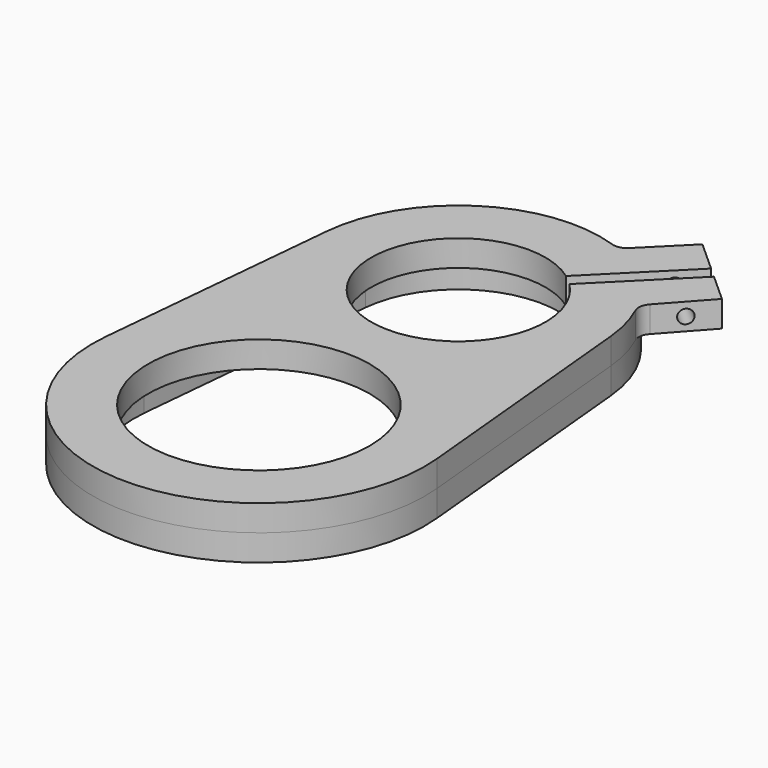
from build123d import *

# Parameters (mm, degrees)
F3_R      = 4.7625
F3_R_2    = 50.8
F4_DEPTH  = 11.9888
F5_R      = 3.175
F6_DEPTH  = 133.893314743
F8_DEPTH  = 11.9888
F10_DEPTH = 6.35
F11_DEPTH = 6.35
F12_DEPTH = 6.35


# Not quite as in the source:
# - a variable given as a bare number and used for a length is read in inches; the dataset says mm whatever the document's units were


with BuildPart() as f4:
    # F3 (on Top) → F4 (new body)
    with BuildSketch(Plane.XY):
        with BuildLine():
            ThreePointArc((28.2843044815, 64.8573104526), (-25.9422769004, 6.1262979516), (23.4354987006, 68.9887607928))
            Line((23.4354987006, 68.9887607928), (60.3862498519, 105.9395119442))
            Line((60.3862498519, 105.9395119442), (46.2066900189, 118.7007204743))
            Line((46.2066900189, 118.7007204743), (27.5367774821, 100.0308079375))
            ThreePointArc((27.5367774821, 100.0308079375), (24.4893412706, 98.3369938712), (21.0069821329, 98.5074297537))
            ThreePointArc((21.0069821329, 98.5074297537), (-35.5438535466, 91.4710990406), (-65.1074486079, 42.7525110788))
            Line((-65.1074486079, 42.7525110788), (-75.8590828523, -70.5270253622))
            ThreePointArc((-75.8590828523, -70.5270253622), (0, -153.9269940288), (75.8590828523, -70.5270253622))
            Line((75.8590828523, -70.5270253622), (65.1074486079, 42.7525110788))
            ThreePointArc((65.1074486079, 42.7525110788), (63.1878642435, 53.4389467972), (59.5267335018, 63.6605334739))
            ThreePointArc((59.5267335018, 63.6605334739), (59.0305262413, 67.2575870183), (60.5864824449, 70.5384430254))
            Line((60.5864824449, 70.5384430254), (78.0995628634, 89.9980240728))
            Line((78.0995628634, 89.9980240728), (65.1127697963, 101.6857757674))
            Line((65.1127697963, 101.6857757674), (28.2843044815, 64.8573104526))
        make_face()
        with Locations((0, -141.2269940288)):
            Circle(F3_R, mode=Mode.SUBTRACT)
        with Locations((-63.215902377, -71.72702014)):
            Circle(F3_R, mode=Mode.SUBTRACT)
        with Locations((0, -77.7269940288)):
            Circle(F3_R_2, mode=Mode.SUBTRACT)
        with Locations((63.215902377, -71.72702014)):
            Circle(F3_R, mode=Mode.SUBTRACT)
        with Locations((-57.8400852547, -15.0872519195)):
            Circle(F3_R, mode=Mode.SUBTRACT)
        with Locations((-52.4642681325, 41.552516301)):
            Circle(F3_R, mode=Mode.SUBTRACT)
        with Locations((57.8400852547, -15.0872519195)):
            Circle(F3_R, mode=Mode.SUBTRACT)
        with Locations((52.700047, 36.5730059712)):
            Circle(F3_R, mode=Mode.SUBTRACT)
        with Locations((-52.4642681325, 41.552516301)):
            Circle(F3_R)
        with Locations((52.700047, 36.5730059712)):
            Circle(F3_R)
        with Locations((57.8400852547, -15.0872519195)):
            Circle(F3_R)
        with Locations((63.215902377, -71.72702014)):
            Circle(F3_R)
        with Locations((0, -141.2269940288)):
            Circle(F3_R)
        with Locations((-63.215902377, -71.72702014)):
            Circle(F3_R)
        with Locations((-57.8400852547, -15.0872519195)):
            Circle(F3_R)
    extrude(amount=F4_DEPTH)

    # F5 (on face) → F6 (cut, through all)
    with BuildSketch(Plane(origin=(-1.6001270702, 1.4400697524, 0), x_dir=(0.6689532824, 0.7433044504, 0), z_dir=(0.7433044504, -0.6689532824, 0))):
        with Locations((106.0509778379, 5.9944)):
            Circle(F5_R)
    extrude(amount=-F6_DEPTH, mode=Mode.SUBTRACT)

    # F3 (on Top) → F10 (cut)
    with BuildSketch(Plane.XY):
        with Locations((-63.215902377, -71.72702014)):
            Circle(F3_R)
        with Locations((0, -141.2269940288)):
            Circle(F3_R)
        with Locations((63.215902377, -71.72702014)):
            Circle(F3_R)
        with Locations((57.8400852547, -15.0872519195)):
            Circle(F3_R)
        with Locations((52.700047, 36.5730059712)):
            Circle(F3_R)
        with Locations((-57.8400852547, -15.0872519195)):
            Circle(F3_R)
        with Locations((-52.4642681325, 41.552516301)):
            Circle(F3_R)
    extrude(amount=F10_DEPTH, mode=Mode.SUBTRACT)


with BuildPart() as f8:
    # F7 (on Top) → F8 (new body)
    with BuildSketch(Plane.XY):
        with BuildLine():
            Line((-65.1074486079, 42.7525110788), (-75.8590828523, -70.5270253622))
            ThreePointArc((-75.8590828523, -70.5270253622), (0, -153.9269940288), (75.8590828523, -70.5270253622))
            Line((75.8590828523, -70.5270253622), (65.1074486079, 42.7525110788))
            ThreePointArc((65.1074486079, 42.7525110788), (0, 101.9730529712), (-65.1074486079, 42.7525110788))
        make_face()
        with BuildLine():
            ThreePointArc((69.5374926147, -71.1270227511), (0, -147.5769940288), (-69.5374926147, -71.1270227511))
            Line((-69.5374926147, -71.1270227511), (-58.7858583702, 42.1525136899))
            ThreePointArc((-58.7858583702, 42.1525136899), (0, 95.6230529712), (58.7858583702, 42.1525136899))
            Line((58.7858583702, 42.1525136899), (69.5374926147, -71.1270227511))
        make_face(mode=Mode.SUBTRACT)
        with BuildLine():
            Line((-58.7858583702, 42.1525136899), (-69.5374926147, -71.1270227511))
            ThreePointArc((-69.5374926147, -71.1270227511), (0, -147.5769940288), (69.5374926147, -71.1270227511))
            Line((69.5374926147, -71.1270227511), (58.7858583702, 42.1525136899))
            ThreePointArc((58.7858583702, 42.1525136899), (0, 95.6230529712), (-58.7858583702, 42.1525136899))
        make_face()
        with BuildLine():
            ThreePointArc((-4.7591501891, -141.0484002788), (-46.9747184236, -120.4543369023), (-63.487789177, -76.4817529209))
            ThreePointArc((-63.487789177, -76.4817529209), (-67.9646903624, -71.3658845431), (-62.7656453711, -66.9858520477))
            Line((-62.7656453711, -66.9858520477), (-58.2872475671, -19.828712888))
            ThreePointArc((-58.2872475671, -19.828712888), (-62.581253338, -14.6369948193), (-57.3867335585, -10.3463787415))
            Line((-57.3867335585, -10.3463787415), (-52.9083353708, 36.8107644583))
            ThreePointArc((-52.9083353708, 36.8107644583), (-57.1937477857, 42.1123631196), (-51.7889763254, 46.2668971962))
            ThreePointArc((-51.7889763254, 46.2668971962), (2.2047304265, 88.8794003864), (51.8738306744, 41.2965644315))
            Line((51.8738306744, 41.2965644315), (51.8771120982, 41.263867768))
            ThreePointArc((51.8771120982, 41.263867768), (55.7629034103, 40.2199659188), (57.462547, 36.5730059712))
            ThreePointArc((57.462547, 36.5730059712), (56.1117723357, 33.2501252204), (52.8256812849, 31.8121633696))
            Line((52.8256812849, 31.8121633696), (57.0609641731, -10.3889142783))
            ThreePointArc((57.0609641731, -10.3889142783), (60.9199263301, -11.4546240552), (62.6025852547, -15.0872519195))
            ThreePointArc((62.6025852547, -15.0872519195), (61.2672791884, -18.3941761689), (58.0101451534, -19.8467146918))
            Line((58.0101451534, -19.8467146918), (62.7412485767, -66.9882323182))
            ThreePointArc((62.7412485767, -66.9882323182), (66.411279313, -68.1955937303), (67.978402377, -71.72702014))
            ThreePointArc((67.978402377, -71.72702014), (66.6782907965, -74.9970771245), (63.487789177, -76.4817529209))
            ThreePointArc((63.487789177, -76.4817529209), (46.9747184236, -120.4543369023), (4.7591501891, -141.0484002788))
            ThreePointArc((4.7591501891, -141.0484002788), (4.7616624736, -141.1376814475), (4.7625, -141.2269940288))
            ThreePointArc((4.7625, -141.2269940288), (-0.0893125814, -145.9886565025), (-4.7591501891, -141.0484002788))
        make_face(mode=Mode.SUBTRACT)
        with BuildLine():
            ThreePointArc((-58.453402377, -71.72702014), (-59.9458453924, -75.1894085595), (-63.487789177, -76.4817529209))
            ThreePointArc((-63.487789177, -76.4817529209), (-46.9747184236, -120.4543369023), (-4.7591501891, -141.0484002788))
            ThreePointArc((-4.7591501891, -141.0484002788), (0, -136.4644940288), (4.7591501891, -141.0484002788))
            ThreePointArc((4.7591501891, -141.0484002788), (46.9747184236, -120.4543369023), (63.487789177, -76.4817529209))
            ThreePointArc((63.487789177, -76.4817529209), (58.4680595012, -72.1003755704), (62.7412485767, -66.9882323182))
            Line((62.7412485767, -66.9882323182), (58.0101451534, -19.8467146918))
            ThreePointArc((58.0101451534, -19.8467146918), (53.1013896487, -15.5628254719), (57.0609641731, -10.3889142783))
            Line((57.0609641731, -10.3889142783), (52.8256812849, 31.8121633696))
            ThreePointArc((52.8256812849, 31.8121633696), (47.961351394, 36.0974324188), (51.8771120982, 41.263867768))
            Line((51.8771120982, 41.263867768), (51.8738306744, 41.2965644315))
            ThreePointArc((51.8738306744, 41.2965644315), (2.2047304265, 88.8794003864), (-51.7889763254, 46.2668971962))
            ThreePointArc((-51.7889763254, 46.2668971962), (-48.8658321194, 44.6722381651), (-47.7017681325, 41.552516301))
            ThreePointArc((-47.7017681325, 41.552516301), (-49.2575146319, 38.0314172912), (-52.9083353708, 36.8107644583))
            Line((-52.9083353708, 36.8107644583), (-57.3867335585, -10.3463787415))
            ThreePointArc((-57.3867335585, -10.3463787415), (-54.3158481952, -11.8839474696), (-53.0775852547, -15.0872519195))
            ThreePointArc((-53.0775852547, -15.0872519195), (-54.63448112, -18.6093973426), (-58.2872475671, -19.828712888))
            Line((-58.2872475671, -19.828712888), (-62.7656453711, -66.9858520477))
            ThreePointArc((-62.7656453711, -66.9858520477), (-59.6927109799, -68.5225656419), (-58.453402377, -71.72702014))
        make_face()
        with BuildLine():
            ThreePointArc((56.8943121393, -72.3270175288), (0, -134.8769940288), (-56.8943121393, -72.3270175288))
            Line((-56.8943121393, -72.3270175288), (-46.1426778948, 40.9525189121))
            ThreePointArc((-46.1426778948, 40.9525189121), (0, 82.9230529712), (46.1426778948, 40.9525189121))
            Line((46.1426778948, 40.9525189121), (56.8943121393, -72.3270175288))
        make_face(mode=Mode.SUBTRACT)
        with BuildLine():
            ThreePointArc((57.0609641731, -10.3889142783), (53.1013896487, -15.5628254719), (58.0101451534, -19.8467146918))
            Line((58.0101451534, -19.8467146918), (57.0609641731, -10.3889142783))
        make_face()
        with BuildLine():
            Line((57.0609641731, -10.3889142783), (58.0101451534, -19.8467146918))
            ThreePointArc((58.0101451534, -19.8467146918), (61.2672791884, -18.3941761689), (62.6025852547, -15.0872519195))
            ThreePointArc((62.6025852547, -15.0872519195), (60.9199263301, -11.4546240552), (57.0609641731, -10.3889142783))
        make_face()
        with BuildLine():
            ThreePointArc((63.1826080799, -71.3860133301), (63.3864261952, -73.9308151341), (63.487789177, -76.4817529209))
            ThreePointArc((63.487789177, -76.4817529209), (66.6782907965, -74.9970771245), (67.978402377, -71.72702014))
            ThreePointArc((67.978402377, -71.72702014), (66.411279313, -68.1955937303), (62.7412485767, -66.9882323182))
            Line((62.7412485767, -66.9882323182), (63.1826080799, -71.3860133301))
        make_face()
        with BuildLine():
            ThreePointArc((62.7412485767, -66.9882323182), (58.4680595012, -72.1003755704), (63.487789177, -76.4817529209))
            ThreePointArc((63.487789177, -76.4817529209), (63.3864261952, -73.9308151341), (63.1826080799, -71.3860133301))
            Line((63.1826080799, -71.3860133301), (62.7412485767, -66.9882323182))
        make_face()
        with BuildLine():
            ThreePointArc((4.7591501891, -141.0484002788), (0, -136.4644940288), (-4.7591501891, -141.0484002788))
            ThreePointArc((-4.7591501891, -141.0484002788), (0, -141.2269940288), (4.7591501891, -141.0484002788))
        make_face()
        with BuildLine():
            ThreePointArc((4.7591501891, -141.0484002788), (0, -141.2269940288), (-4.7591501891, -141.0484002788))
            ThreePointArc((-4.7591501891, -141.0484002788), (-0.0893125814, -145.9886565025), (4.7625, -141.2269940288))
            ThreePointArc((4.7625, -141.2269940288), (4.7616624736, -141.1376814475), (4.7591501891, -141.0484002788))
        make_face()
        with BuildLine():
            Line((-62.7656453711, -66.9858520477), (-63.2155744434, -71.723566026))
            ThreePointArc((-63.2155744434, -71.723566026), (-63.3963380158, -74.1001047026), (-63.487789177, -76.4817529209))
            ThreePointArc((-63.487789177, -76.4817529209), (-59.9458453924, -75.1894085595), (-58.453402377, -71.72702014))
            ThreePointArc((-58.453402377, -71.72702014), (-59.6927109799, -68.5225656419), (-62.7656453711, -66.9858520477))
        make_face()
        with BuildLine():
            ThreePointArc((-63.487789177, -76.4817529209), (-63.3963380158, -74.1001047026), (-63.2155744434, -71.723566026))
            Line((-63.2155744434, -71.723566026), (-62.7656453711, -66.9858520477))
            ThreePointArc((-62.7656453711, -66.9858520477), (-67.9646903624, -71.3658845431), (-63.487789177, -76.4817529209))
        make_face()
        with BuildLine():
            Line((-57.3867335585, -10.3463787415), (-58.2872475671, -19.828712888))
            ThreePointArc((-58.2872475671, -19.828712888), (-54.63448112, -18.6093973426), (-53.0775852547, -15.0872519195))
            ThreePointArc((-53.0775852547, -15.0872519195), (-54.3158481952, -11.8839474696), (-57.3867335585, -10.3463787415))
        make_face()
        with BuildLine():
            ThreePointArc((-57.3867335585, -10.3463787415), (-62.581253338, -14.6369948193), (-58.2872475671, -19.828712888))
            Line((-58.2872475671, -19.828712888), (-57.3867335585, -10.3463787415))
        make_face()
        with BuildLine():
            ThreePointArc((-51.7889763254, 46.2668971962), (-57.1937477857, 42.1123631196), (-52.9083353708, 36.8107644583))
            Line((-52.9083353708, 36.8107644583), (-52.4933051133, 41.1809969535))
            ThreePointArc((-52.4933051133, 41.1809969535), (-52.2034780379, 43.7325799552), (-51.7889763254, 46.2668971962))
        make_face()
        with BuildLine():
            Line((-52.4933051133, 41.1809969535), (-52.9083353708, 36.8107644583))
            ThreePointArc((-52.9083353708, 36.8107644583), (-49.2575146319, 38.0314172912), (-47.7017681325, 41.552516301))
            ThreePointArc((-47.7017681325, 41.552516301), (-48.8658321194, 44.6722381651), (-51.7889763254, 46.2668971962))
            ThreePointArc((-51.7889763254, 46.2668971962), (-52.2034780379, 43.7325799552), (-52.4933051133, 41.1809969535))
        make_face()
        with BuildLine():
            ThreePointArc((57.462547, 36.5730059712), (55.7629034103, 40.2199659188), (51.8771120982, 41.263867768))
            Line((51.8771120982, 41.263867768), (52.8256812849, 31.8121633696))
            ThreePointArc((52.8256812849, 31.8121633696), (56.1117723357, 33.2501252204), (57.462547, 36.5730059712))
        make_face()
        with BuildLine():
            Line((52.8256812849, 31.8121633696), (51.8771120982, 41.263867768))
            ThreePointArc((51.8771120982, 41.263867768), (47.961351394, 36.0974324188), (52.8256812849, 31.8121633696))
        make_face()
    extrude(amount=-F8_DEPTH)

    # F9 (on face) → F11 (cut)
    with BuildSketch(Plane(origin=(0, 0, -11.9888), x_dir=(1, 0, 0), z_dir=(0, 0, -1))):
        with BuildLine():
            Line((-69.5374926147, 71.1270227511), (-58.7858583702, -42.1525136899))
            ThreePointArc((-58.7858583702, -42.1525136899), (0, -95.6230529712), (58.7858583702, -42.1525136899))
            Line((58.7858583702, -42.1525136899), (69.5374926147, 71.1270227511))
            ThreePointArc((69.5374926147, 71.1270227511), (0, 147.5769940288), (-69.5374926147, 71.1270227511))
        make_face()
        with BuildLine():
            Line((-52.4933051133, -41.1809969535), (-63.2155744434, 71.723566026))
            ThreePointArc((-63.2155744434, 71.723566026), (0.1695793351, 141.2267675942), (63.1826080799, 71.3860133301))
            Line((63.1826080799, 71.3860133301), (51.8738306744, -41.2965644315))
            ThreePointArc((51.8738306744, -41.2965644315), (-0.3625570138, -88.9394898731), (-52.4933051133, -41.1809969535))
        make_face(mode=Mode.SUBTRACT)
    extrude(amount=-F11_DEPTH, mode=Mode.SUBTRACT)

    # F7 (on Top) → F12 (cut)
    with BuildSketch(Plane.XY):
        with BuildLine():
            ThreePointArc((62.7412485767, -66.9882323182), (58.4680595012, -72.1003755704), (63.487789177, -76.4817529209))
            ThreePointArc((63.487789177, -76.4817529209), (63.3864261952, -73.9308151341), (63.1826080799, -71.3860133301))
            Line((63.1826080799, -71.3860133301), (62.7412485767, -66.9882323182))
        make_face()
        with BuildLine():
            ThreePointArc((63.1826080799, -71.3860133301), (63.3864261952, -73.9308151341), (63.487789177, -76.4817529209))
            ThreePointArc((63.487789177, -76.4817529209), (66.6782907965, -74.9970771245), (67.978402377, -71.72702014))
            ThreePointArc((67.978402377, -71.72702014), (66.411279313, -68.1955937303), (62.7412485767, -66.9882323182))
            Line((62.7412485767, -66.9882323182), (63.1826080799, -71.3860133301))
        make_face()
        with BuildLine():
            ThreePointArc((57.0609641731, -10.3889142783), (53.1013896487, -15.5628254719), (58.0101451534, -19.8467146918))
            Line((58.0101451534, -19.8467146918), (57.0609641731, -10.3889142783))
        make_face()
        with BuildLine():
            Line((57.0609641731, -10.3889142783), (58.0101451534, -19.8467146918))
            ThreePointArc((58.0101451534, -19.8467146918), (61.2672791884, -18.3941761689), (62.6025852547, -15.0872519195))
            ThreePointArc((62.6025852547, -15.0872519195), (60.9199263301, -11.4546240552), (57.0609641731, -10.3889142783))
        make_face()
        with BuildLine():
            Line((52.8256812849, 31.8121633696), (51.8771120982, 41.263867768))
            ThreePointArc((51.8771120982, 41.263867768), (47.961351394, 36.0974324188), (52.8256812849, 31.8121633696))
        make_face()
        with BuildLine():
            ThreePointArc((57.462547, 36.5730059712), (55.7629034103, 40.2199659188), (51.8771120982, 41.263867768))
            Line((51.8771120982, 41.263867768), (52.8256812849, 31.8121633696))
            ThreePointArc((52.8256812849, 31.8121633696), (56.1117723357, 33.2501252204), (57.462547, 36.5730059712))
        make_face()
        with BuildLine():
            Line((-52.4933051133, 41.1809969535), (-52.9083353708, 36.8107644583))
            ThreePointArc((-52.9083353708, 36.8107644583), (-49.2575146319, 38.0314172912), (-47.7017681325, 41.552516301))
            ThreePointArc((-47.7017681325, 41.552516301), (-48.8658321194, 44.6722381651), (-51.7889763254, 46.2668971962))
            ThreePointArc((-51.7889763254, 46.2668971962), (-52.2034780379, 43.7325799552), (-52.4933051133, 41.1809969535))
        make_face()
        with BuildLine():
            ThreePointArc((-51.7889763254, 46.2668971962), (-57.1937477857, 42.1123631196), (-52.9083353708, 36.8107644583))
            Line((-52.9083353708, 36.8107644583), (-52.4933051133, 41.1809969535))
            ThreePointArc((-52.4933051133, 41.1809969535), (-52.2034780379, 43.7325799552), (-51.7889763254, 46.2668971962))
        make_face()
        with BuildLine():
            Line((-57.3867335585, -10.3463787415), (-58.2872475671, -19.828712888))
            ThreePointArc((-58.2872475671, -19.828712888), (-54.63448112, -18.6093973426), (-53.0775852547, -15.0872519195))
            ThreePointArc((-53.0775852547, -15.0872519195), (-54.3158481952, -11.8839474696), (-57.3867335585, -10.3463787415))
        make_face()
        with BuildLine():
            ThreePointArc((-57.3867335585, -10.3463787415), (-62.581253338, -14.6369948193), (-58.2872475671, -19.828712888))
            Line((-58.2872475671, -19.828712888), (-57.3867335585, -10.3463787415))
        make_face()
        with BuildLine():
            Line((-62.7656453711, -66.9858520477), (-63.2155744434, -71.723566026))
            ThreePointArc((-63.2155744434, -71.723566026), (-63.3963380158, -74.1001047026), (-63.487789177, -76.4817529209))
            ThreePointArc((-63.487789177, -76.4817529209), (-59.9458453924, -75.1894085595), (-58.453402377, -71.72702014))
            ThreePointArc((-58.453402377, -71.72702014), (-59.6927109799, -68.5225656419), (-62.7656453711, -66.9858520477))
        make_face()
        with BuildLine():
            ThreePointArc((-63.487789177, -76.4817529209), (-63.3963380158, -74.1001047026), (-63.2155744434, -71.723566026))
            Line((-63.2155744434, -71.723566026), (-62.7656453711, -66.9858520477))
            ThreePointArc((-62.7656453711, -66.9858520477), (-67.9646903624, -71.3658845431), (-63.487789177, -76.4817529209))
        make_face()
        with BuildLine():
            ThreePointArc((4.7591501891, -141.0484002788), (0, -136.4644940288), (-4.7591501891, -141.0484002788))
            ThreePointArc((-4.7591501891, -141.0484002788), (0, -141.2269940288), (4.7591501891, -141.0484002788))
        make_face()
        with BuildLine():
            ThreePointArc((4.7591501891, -141.0484002788), (0, -141.2269940288), (-4.7591501891, -141.0484002788))
            ThreePointArc((-4.7591501891, -141.0484002788), (-0.0893125814, -145.9886565025), (4.7625, -141.2269940288))
            ThreePointArc((4.7625, -141.2269940288), (4.7616624736, -141.1376814475), (4.7591501891, -141.0484002788))
        make_face()
    extrude(amount=-F12_DEPTH, mode=Mode.SUBTRACT)


solid = Compound([f4.part, f8.part])
